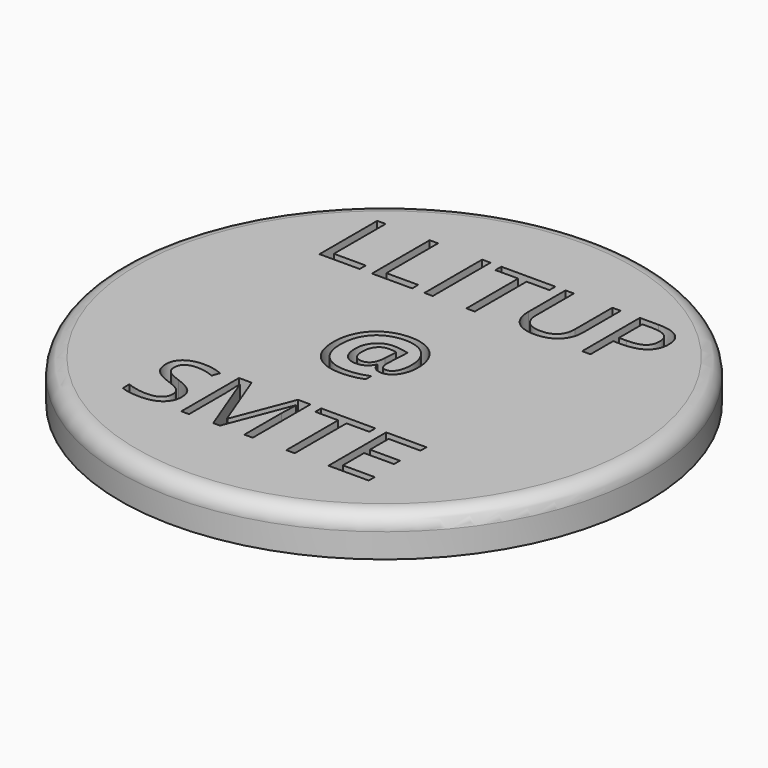
from build123d import *

# Parameters (mm, degrees)
F0_R         = 32.5
F1_DEPTH     = 5
F2_TEXT_SIZE = 12.4465188643
F3_DEPTH     = 5.001
F4_R         = 2


# Not quite as in the source:
# - Text() gives the source's letters only with a copy of the font that has no kerning and outlines rounded to 1/6400 em; it was checked with that copy


with BuildPart() as f1:
    # F0 (on Top) → F1 (new body)
    with BuildSketch(Plane.XY):
        Circle(F0_R)
    extrude(amount=F1_DEPTH)

    # F2 (on face) → F3 (cut, through all)
    with BuildSketch(Plane.XY.offset(5)):
        with Locations((-19.4866113614, 12.8874602534)):
            Text('LLITUP', F2_TEXT_SIZE, font='Open Sans', text_align=(TextAlign.LEFT, TextAlign.BOTTOM))
        with Locations((-6.5500108169, -4.039805402)):
            Text('@', F2_TEXT_SIZE, font='Open Sans', text_align=(TextAlign.LEFT, TextAlign.BOTTOM))
        with Locations((-16.2524612253, -20.9670710574)):
            Text('SMTE', F2_TEXT_SIZE, font='Open Sans', text_align=(TextAlign.LEFT, TextAlign.BOTTOM))
    extrude(amount=-F3_DEPTH, mode=Mode.SUBTRACT)

    # F4
    f4_edges = [f1.edges().sort_by_distance(p)[0] for p in [
        (-32.5, 0, 5),
    ]]
    fillet(f4_edges, radius=F4_R)


solid = f1.part
